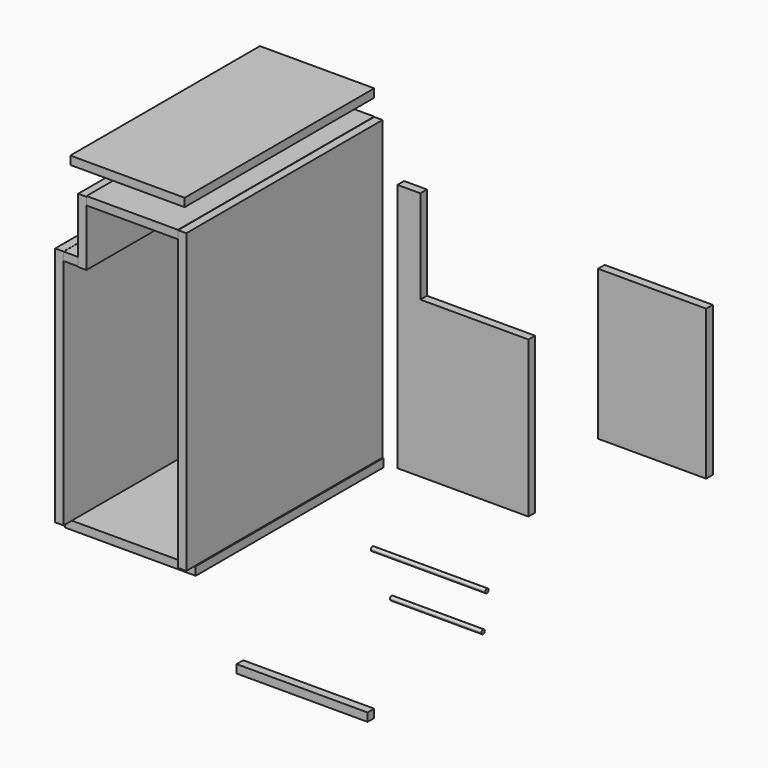
from build123d import *

# Parameters (mm, degrees)
F1_DEPTH  = 2
F2_W      = 2
F2_H      = 15.5
F3_DEPTH  = 59
F4_W      = 3.5
F4_H      = 2
F5_DEPTH  = 59
F6_W      = 2
F6_H      = 71.5
F7_DEPTH  = 59
F8_W      = 2
F8_H      = 58
F9_DEPTH  = 59
F10_W     = 22
F10_H     = 2
F11_DEPTH = 59
F12_W     = 31.5
F12_H     = 2
F13_DEPTH = 56.5
F14_W     = 27.5
F14_H     = 2
F15_DEPTH = 57
F17_DEPTH = 2
F18_W     = 27.5
F18_H     = 33.5
F19_DEPTH = 2
F20_W     = 26
F20_H     = 36
F21_DEPTH = 2
F22_W     = 27.5
F22_H     = 1
F23_DEPTH = 1
F24_R     = 0.49999
F25_W     = 22
F25_H     = 1
F26_DEPTH = 1
F27_R     = 0.49999
F28_W     = 31.5
F28_H     = 2
F29_DEPTH = 2


# Not quite as in the source:
# - a fillet or chamfer is up to 0.001 mm smaller than in the source, because OpenCascade refuses the exact size


with BuildPart() as f1:
    # F0 (on Front) → F1 (new body)
    with BuildSketch(Plane.XZ):
        Polygon((-22, 43.0476225019), (-27.5, 43.0476225019), (-27.5, -12.9523774981), (0, -12.9523774981), (0, 56.5476225019), (-22, 56.5476225019), align=None)
    extrude(amount=F1_DEPTH)


with BuildPart() as f3:
    # F2 (on Front) → F3 (new body)
    with BuildSketch(Plane.XZ):
        with Locations((-23.0228824764, 50.7314585745)):
            Rectangle(F2_W, F2_H)
    extrude(amount=F3_DEPTH)


with BuildPart() as f5:
    # F4 (on Front) → F5 (new body)
    with BuildSketch(Plane.XZ):
        with Locations((-25.7554331869, 44.1044030488)):
            Rectangle(F4_W, F4_H)
    extrude(amount=F5_DEPTH)


with BuildPart() as f7:
    # F6 (on Front) → F7 (new body)
    with BuildSketch(Plane.XZ):
        with Locations((1, 22.834235996)):
            Rectangle(F6_W, F6_H)
    extrude(amount=F7_DEPTH)


with BuildPart() as f9:
    # F8 (on Front) → F9 (new body)
    with BuildSketch(Plane.XZ):
        with Locations((-28.5317020714, 16.1130948886)):
            Rectangle(F8_W, F8_H)
    extrude(amount=F9_DEPTH)


with BuildPart() as f11:
    # F10 (on Front) → F11 (new body)
    with BuildSketch(Plane.XZ):
        with Locations((-11, 57.6625595093)):
            Rectangle(F10_W, F10_H)
    extrude(amount=F11_DEPTH)


with BuildPart() as f13:
    # F12 (on Front) → F13 (new body)
    with BuildSketch(Plane.XZ):
        with Locations((-13.4842316415, -13.8856245428)):
            Rectangle(F12_W, F12_H)
    extrude(amount=F13_DEPTH)


with BuildPart() as f15:
    # F14 (on Front) → F15 (new body)
    with BuildSketch(Plane.XZ):
        with Locations((-13.75, 63.635656774)):
            Rectangle(F14_W, F14_H)
    extrude(amount=F15_DEPTH)


with BuildPart() as f17:
    # F16 (on Front) → F17 (new body)
    with BuildSketch(Plane.XZ):
        Polygon((7.1751703918, 24.8444598615), (7.1751703918, -12.6555401385), (38.6751703918, -12.6555401385), (38.6751703918, 24.8444598615), (12.6751703918, 24.8444598615), (12.6751703918, 47.3444598615), (7.1751703918, 47.3444598615), align=None)
    extrude(amount=F17_DEPTH)


with BuildPart() as f19:
    # F18 (on Front) → F19 (new body)
    with BuildSketch(Plane.XZ):
        with Locations((-45.5933791399, -19.8420215845)):
            Rectangle(F18_W, F18_H)
    extrude(amount=F19_DEPTH)


with BuildPart() as f21:
    # F20 (on Front) → F21 (new body)
    with BuildSketch(Plane.XZ):
        with Locations((68.4304798841, 27.2750734985)):
            Rectangle(F20_W, F20_H)
    extrude(amount=F21_DEPTH)


with BuildPart() as f23:
    # F22 (on Front) → F23 (new body)
    with BuildSketch(Plane.XZ):
        with Locations((13.75, -32.6339128315)):
            Rectangle(F22_W, F22_H)
    extrude(amount=F23_DEPTH)

    # F24 (radius 0.5 in the source; OpenCascade refuses exactly that, so slightly less here)
    f24_edges = [f23.edges().sort_by_distance(p)[0] for p in [
        (13.75, -1, -33.133913),
        (13.75, -1, -32.133913),
        (13.75, 0, -33.133913),
        (13.75, 0, -32.133913),
    ]]
    fillet(f24_edges, radius=F24_R)


with BuildPart() as f26:
    # F25 (on Front) → F26 (new body)
    with BuildSketch(Plane.XZ):
        with Locations((15.5834236741, -41.5960076153)):
            Rectangle(F25_W, F25_H)
    extrude(amount=F26_DEPTH)

    # F27 (radius 0.5 in the source; OpenCascade refuses exactly that, so slightly less here)
    f27_edges = [f26.edges().sort_by_distance(p)[0] for p in [
        (15.583424, -1, -41.096008),
        (15.583424, -1, -42.096008),
        (15.583424, 0, -42.096008),
        (15.583424, 0, -41.096008),
    ]]
    fillet(f27_edges, radius=F27_R)


with BuildPart() as f29:
    # F28 (on Front) → F29 (new body)
    with BuildSketch(Plane.XZ):
        with Locations((-15.75, -67.7069892883)):
            Rectangle(F28_W, F28_H)
    extrude(amount=F29_DEPTH)


solid = Compound([f1.part, f3.part, f5.part, f7.part, f9.part, f11.part, f13.part, f15.part, f17.part, f19.part, f21.part, f23.part, f26.part, f29.part])
